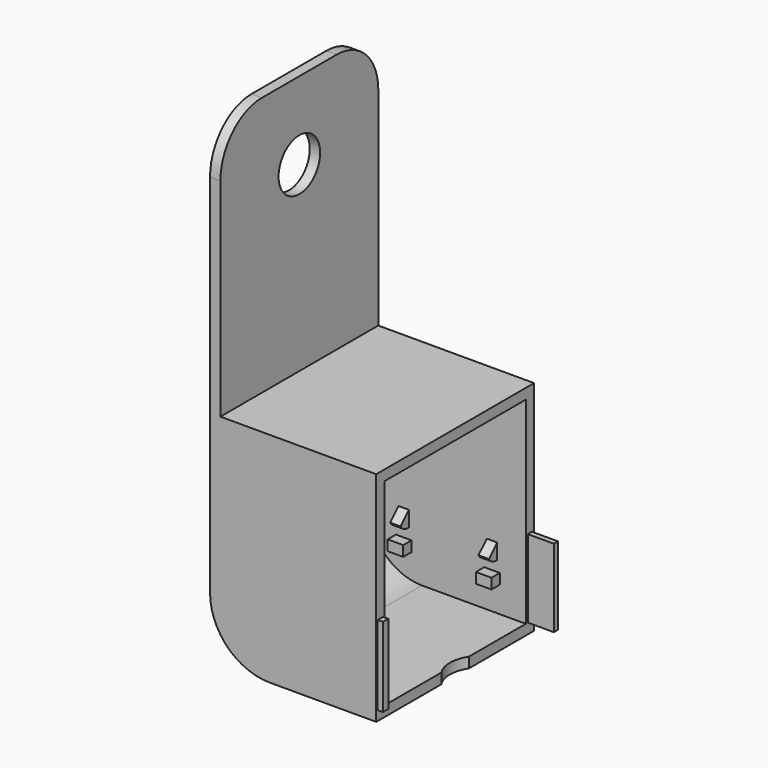
from build123d import *

# Parameters (mm, degrees)
F1_DEPTH     = 38
F3_D         = 12
F4_R         = 10
F6_D         = 10
F8_DEPTH     = 2
F10_DEPTH    = 2
F11_W        = 30
F11_H        = 38
F12_DEPTH    = 2
F14_W        = 1
F14_H        = 15
F15_DEPTH    = 5
F16_W        = 2
F16_H        = 3
F18_DEPTH    = 2
F17_W        = 2
F17_H        = 3
F19_DEPTH    = 2
F20_SIZE     = 1.99999
F21_T1_DEPTH = 10.6602829052
F21_T3_DEPTH = 10.6602829052
F14_W_2      = 1.3
F14_H_2      = 15.3
F22_DEPTH    = 1


# Not quite as in the source:
# - a fillet or chamfer that OpenCascade refuses, or shapes differently, is made with other operations: its cross-section is extruded or revolved along the edge and cut away or added
# - a fillet or chamfer is up to 0.001 mm smaller than in the source, because OpenCascade refuses the exact size
# - a feature names something its author has since deleted; it is built from what else it names


with BuildPart() as f1:
    # F0 (on Front) → F1 (new body)
    with BuildSketch(Plane.XZ):
        with BuildLine():
            Line((-30, 90), (-32, 90))
            Line((-32, 90), (-32, 9.5))
            ThreePointArc((-32, 9.5), (-28.6317279836, 1.3682720164), (-20.5, -2))
            Line((-20.5, -2), (0, -2))
            Line((0, -2), (0, 0))
            Line((0, 0), (-20, 0))
            ThreePointArc((-20, 0), (-27.0710678119, 2.9289321881), (-30, 10))
            Line((-30, 10), (-30, 90))
        make_face()
    extrude(amount=F1_DEPTH)

    # F3 (through all)
    with Locations(Plane.XY):
        with Locations((5, -19)):
            Hole(F3_D / 2)

    # F4
    f4_edges = [f1.edges().sort_by_distance(p)[0] for p in [
        (-31, -38, 90),
        (-31, 0, 90),
    ]]
    fillet(f4_edges, radius=F4_R)

    # F6 (through all)
    with Locations(Plane.YZ.offset(-30)):
        with Locations((-19, 75)):
            Hole(F6_D / 2)

    # F7 (on face) → F8 (join)
    with BuildSketch(Plane.XZ.offset(38)):
        with BuildLine():
            Line((-20, 0), (0, 0))
            Line((0, 0), (0, 40))
            Line((0, 40), (-30, 40))
            Line((-30, 40), (-30, 10))
            ThreePointArc((-30, 10), (-27.0710678119, 2.9289321881), (-20, 0))
        make_face()
    extrude(amount=-F8_DEPTH)

    # F9 (on face) → F10 (join)
    with BuildSketch(Plane(origin=(0, 0, 0), x_dir=(-1, 0, 0), z_dir=(0, 1, 0))):
        with BuildLine():
            Line((0, 40), (0, 0))
            Line((0, 0), (20, 0))
            ThreePointArc((20, 0), (27.0710678119, 2.9289321881), (30, 10))
            Line((30, 10), (30, 40))
            Line((30, 40), (0, 40))
        make_face()
    extrude(amount=-F10_DEPTH)

    # F11 (on face) → F12 (join)
    with BuildSketch(Plane.XY.offset(40)):
        with Locations((-15, -19)):
            Rectangle(F11_W, F11_H)
    extrude(amount=-F12_DEPTH)

    # F13: union 

    # F14 (on face) → F15 (join)
    with BuildSketch(Plane.YZ):
        with Locations((-1, 7.5)):
            Rectangle(F14_W, F14_H)
    extrude(amount=F15_DEPTH)

    # F16 (on face) → F18 (join)
    with BuildSketch(Plane.XZ.offset(2)):
        with Locations((-6.5, 10.5)):
            Rectangle(F16_W, F16_H)
        Polygon((-5, 5), (-5, 6), (-5, 7), (-8, 7), (-8, 5), align=None)
        with Locations((-23.5, 10.5)):
            Rectangle(F16_W, F16_H)
        Polygon((-25, 7), (-25, 6), (-25, 5), (-22, 5), (-22, 7), align=None)
    extrude(amount=F18_DEPTH)

    # F17 (on face) → F19 (join)
    with BuildSketch(Plane(origin=(0, -36, 0), x_dir=(-1, 0, 0), z_dir=(0, 1, 0))):
        with Locations((6.5, 10.5)):
            Rectangle(F17_W, F17_H)
        Polygon((5, 7), (5, 6), (5, 5), (8, 5), (8, 7), align=None)
        Polygon((25, 5), (25, 6), (25, 7), (22, 7), (22, 5), align=None)
        with Locations((23.5, 10.5)):
            Rectangle(F17_W, F17_H)
    extrude(amount=F19_DEPTH)

    # F20 (size 2 in the source; OpenCascade refuses exactly that, so slightly less here)
    f20_edges = [f1.edges().sort_by_distance(p)[0] for p in [
        (-6.5, -34, 12),
        (-23.5, -34, 12),
        (-6.5, -4, 12),
        (-23.5, -4, 12),
    ]]
    chamfer(f20_edges, length=F20_SIZE)

    # F21: fillet of radius 2 on 4 edges, made by hand

    # F21_s2 → F21_t1 (cut)
    with BuildSketch(Plane.YZ.offset(-11.8301414526)):
        with BuildLine():
            ThreePointArc((-35.732056581, 9), (-34.732051581, 9.2679520792), (-34, 10.00001))
            Line((-34, 10.00001), (-34, 9))
            Line((-34, 9), (-35.732056581, 9))
        make_face()
        with BuildLine():
            ThreePointArc((-2.267943419, 9), (-3.267948419, 9.2679520792), (-4, 10.00001))
            Line((-4, 10.00001), (-4, 9))
            Line((-4, 9), (-2.267943419, 9))
        make_face()
    extrude(amount=F21_T1_DEPTH, mode=Mode.SUBTRACT)

    # F21_s4 → F21_t3 (cut)
    with BuildSketch(Plane.YZ.offset(-28.8301414526)):
        with BuildLine():
            ThreePointArc((-34, 10.00001), (-34.732051581, 9.2679520792), (-35.732056581, 9))
            Line((-35.732056581, 9), (-34, 9))
            Line((-34, 9), (-34, 10.00001))
        make_face()
        with BuildLine():
            ThreePointArc((-2.267943419, 9), (-3.267948419, 9.2679520792), (-4, 10.00001))
            Line((-4, 10.00001), (-4, 9))
            Line((-4, 9), (-2.267943419, 9))
        make_face()
    extrude(amount=F21_T3_DEPTH, mode=Mode.SUBTRACT)

    # F14 (on face) → F22 (join)
    with BuildSketch(Plane.YZ):
        with Locations((-37, 7.5)):
            Rectangle(F14_W_2, F14_H_2)
    extrude(amount=F22_DEPTH)


solid = f1.part
